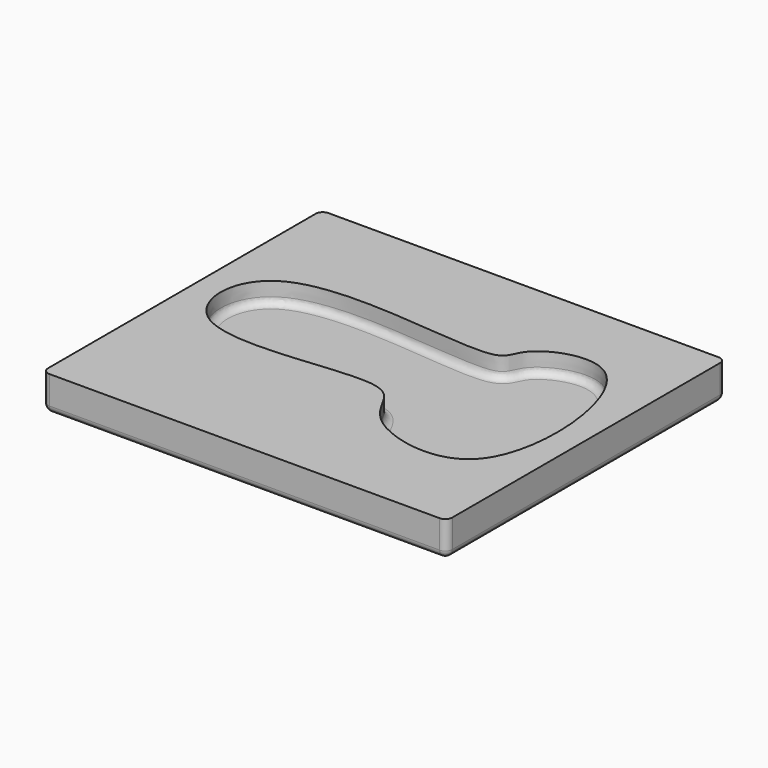
from build123d import *

# Parameters (mm, degrees)
F0_W         = 57.545196265
F0_H         = 49.6331304312
F1_DEPTH     = 5
F3_DEPTH     = 3
F4_R         = 1
F5_R         = 1
F6_T1_DEPTH  = 6.5
F6_S5_W      = 1
F6_S5_H      = 1
F6_T6_DEPTH  = 1
F6_S11_W     = 1
F6_S11_H     = 1
F6_T12_DEPTH = 1
F6_S17_W     = 1
F6_S17_H     = 1
F6_T18_DEPTH = 1
F6_S23_W     = 1
F6_S23_H     = 1
F6_T24_DEPTH = 1


# Not quite as in the source:
# - a fillet or chamfer that OpenCascade refuses, or shapes differently, is made with other operations: its cross-section is extruded or revolved along the edge and cut away or added


with BuildPart() as f1:
    # F0 (on Top) → F1 (new body)
    with BuildSketch(Plane.XY):
        with Locations((-28.7725981325, 24.8165652156)):
            Rectangle(F0_W, F0_H)
    extrude(amount=F1_DEPTH)

    # F2 (on face) → F3 (cut)
    with BuildSketch(Plane.XY.offset(5)):
        with BuildLine():
            add(Edge.make_bspline(
                [(-50.7095903158, 33.3512835205), (-43.7013698504, 37.8214274221), (-18.673590368, 31.614362599), (-19.7404428015, 38.1722724367), (-4.1654089796, 44.5314003001), (-1.0282642758, 9.0887494889), (-19.0832171907, 11.9451255403), (-23.0886976429, 16.7013972458), (-25.4208773961, 23.3690335903), (-54.7670247126, 14.9266655159), (-55.1242446077, 30.5354274757), (-50.7095903158, 33.3512835205)],
                knots=[0, 0, 0, 0, 0.1702800108, 0.2303210763, 0.3285828559, 0.4832861562, 0.5921776589, 0.6687943458, 0.7388292511, 0.8927363395, 1, 1, 1, 1], degree=3))
        make_face()
    extrude(amount=-F3_DEPTH, mode=Mode.SUBTRACT)

    # F4
    f4_edges = [f1.edges().sort_by_distance(p)[0] for p in [
        (-4.545372, 17.775256, 2),
    ]]
    fillet(f4_edges, radius=F4_R)

    # F5
    f5_edges = [f1.edges().sort_by_distance(p)[0] for p in [
        (-57.545196, 24.816565, 0),
        (-28.772598, 0, 0),
        (0, 24.816565, 0),
        (-28.772598, 49.63313, 0),
    ]]
    fillet(f5_edges, radius=F5_R)

    # F6: fillet of radius 1 on 4 edges, made by hand

    # F6_s2 → F6_t1 (cut)
    with BuildSketch(Plane.XY.offset(1)):
        with BuildLine():
            ThreePointArc((-57.545196265, 48.6331304312), (-57.2523030462, 49.3402372124), (-56.545196265, 49.6331304312))
            Line((-56.545196265, 49.6331304312), (-57.545196265, 49.6331304312))
            Line((-57.545196265, 49.6331304312), (-57.545196265, 48.6331304312))
        make_face()
        with BuildLine():
            ThreePointArc((-1, 0), (-0.2928932188, 0.2928932188), (0, 1))
            Line((0, 1), (0, 0))
            Line((0, 0), (-1, 0))
        make_face()
        with BuildLine():
            ThreePointArc((-1, 49.6331304312), (-0.2928932188, 49.3402372124), (0, 48.6331304312))
            Line((0, 48.6331304312), (0, 49.6331304312))
            Line((0, 49.6331304312), (-1, 49.6331304312))
        make_face()
        with BuildLine():
            ThreePointArc((-57.545196265, 1), (-57.2523030462, 0.2928932188), (-56.545196265, 0))
            Line((-56.545196265, 0), (-57.545196265, 0))
            Line((-57.545196265, 0), (-57.545196265, 1))
        make_face()
    extrude(amount=F6_T1_DEPTH, mode=Mode.SUBTRACT)


with BuildPart() as f6_tool4:
    # F6_s5 → F6_t6 (new body)
    with BuildSketch(Plane.YZ.offset(-56.545196265)):
        with Locations((0.5, 0.5)):
            Rectangle(F6_S5_W, F6_S5_H)
    extrude(amount=-F6_T6_DEPTH)

    # F6_s7 → F6_t8 (revolve, cut)
    with BuildSketch(Plane(origin=(-56.545196265, 1, 1), x_dir=(0, 0.7071067812, 0.7071067812), z_dir=(0, -0.7071067812, 0.7071067812))):
        with BuildLine():
            ThreePointArc((0, -1), (1, 0), (0, 1))
            Line((0, 1), (0, -1))
        make_face()
    revolve(axis=Axis((-56.545196265, 1, 1), (-1, 0, 0)), mode=Mode.SUBTRACT)


with BuildPart() as f1_1:
    add(f1.part)

    # F6_t3: cut F6_tool4
    add(f6_tool4.part, mode=Mode.SUBTRACT)


with BuildPart() as f6_tool10:
    # F6_s11 → F6_t12 (new body)
    with BuildSketch(Plane.XZ.offset(-48.6331304312)):
        with Locations((-0.5, 0.5)):
            Rectangle(F6_S11_W, F6_S11_H)
    extrude(amount=-F6_T12_DEPTH)

    # F6_s13 → F6_t14 (revolve, cut)
    with BuildSketch(Plane(origin=(-1, 48.6331304312, 1), x_dir=(-0.7071067812, 0, 0.7071067812), z_dir=(-0.7071067812, 0, -0.7071067812))):
        with BuildLine():
            ThreePointArc((0, -1), (1, 0), (0, 1))
            Line((0, 1), (0, -1))
        make_face()
    revolve(axis=Axis((-1, 48.6331304312, 1), (0, 1, 0)), mode=Mode.SUBTRACT)


with BuildPart() as f1_2:
    add(f1_1.part)

    # F6_t9: cut F6_tool10
    add(f6_tool10.part, mode=Mode.SUBTRACT)


with BuildPart() as f6_tool16:
    # F6_s17 → F6_t18 (new body)
    with BuildSketch(Plane.XZ.offset(-1)):
        with Locations((-0.5, 0.5)):
            Rectangle(F6_S17_W, F6_S17_H)
    extrude(amount=F6_T18_DEPTH)

    # F6_s19 → F6_t20 (revolve, cut)
    with BuildSketch(Plane(origin=(-1, 1, 1), x_dir=(-0.7071067812, 0, 0.7071067812), z_dir=(0.7071067812, 0, 0.7071067812))):
        with BuildLine():
            ThreePointArc((0, -1), (1, 0), (0, 1))
            Line((0, 1), (0, -1))
        make_face()
    revolve(axis=Axis((-1, 1, 1), (0, -1, 0)), mode=Mode.SUBTRACT)


with BuildPart() as f1_3:
    add(f1_2.part)

    # F6_t15: cut F6_tool16
    add(f6_tool16.part, mode=Mode.SUBTRACT)


with BuildPart() as f6_tool22:
    # F6_s23 → F6_t24 (new body)
    with BuildSketch(Plane.YZ.offset(-56.545196265)):
        with Locations((49.1331304312, 0.5)):
            Rectangle(F6_S23_W, F6_S23_H)
    extrude(amount=-F6_T24_DEPTH)

    # F6_s25 → F6_t26 (revolve, cut)
    with BuildSketch(Plane(origin=(-56.545196265, 48.6331304312, 1), x_dir=(0, -0.7071067812, 0.7071067812), z_dir=(0, -0.7071067812, -0.7071067812))):
        with BuildLine():
            ThreePointArc((0, -1), (1, 0), (0, 1))
            Line((0, 1), (0, -1))
        make_face()
    revolve(axis=Axis((-56.545196265, 48.6331304312, 1), (-1, 0, 0)), mode=Mode.SUBTRACT)


with BuildPart() as f1_4:
    add(f1_3.part)

    # F6_t21: cut F6_tool22
    add(f6_tool22.part, mode=Mode.SUBTRACT)


solid = f1_4.part
